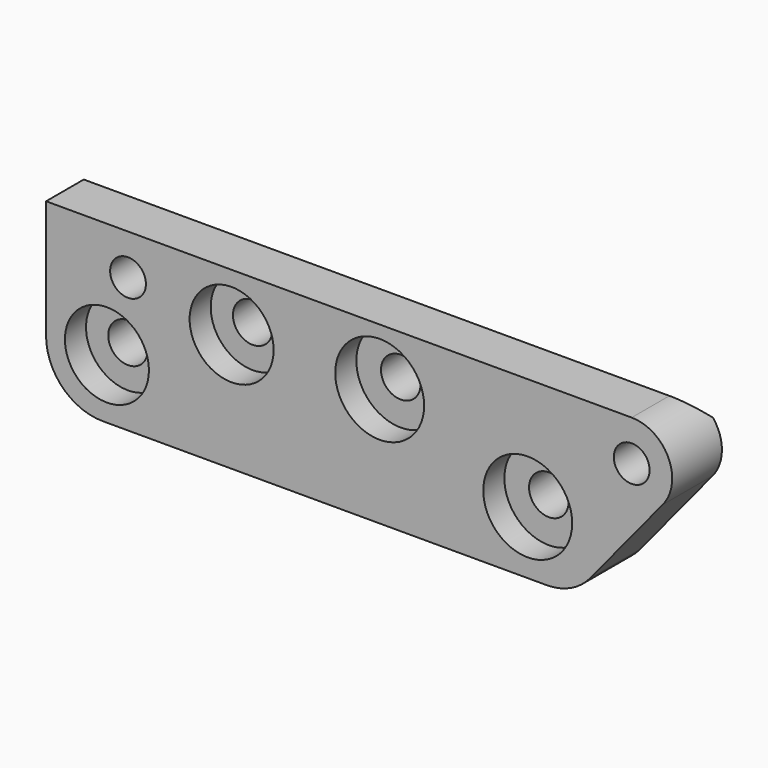
from build123d import *

# Parameters (mm, degrees)
F0_R        = 5.25
F0_R_2      = 4.75
F1_DEPTH    = 16.5
F2_R        = 11.15
F2_R_2      = 11.7991480977
F3_DEPTH    = 7
F4_R        = 15
F5_R        = 15
F6_T1_DEPTH = 176.0234639037


# Not quite as in the source:
# - a fillet or chamfer that OpenCascade refuses, or shapes differently, is made with other operations: its cross-section is extruded or revolved along the edge and cut away or added


with BuildPart() as f1:
    # F0 (on Front) → F1 (new body)
    with BuildSketch(Plane.XZ):
        with BuildLine():
            Line((28.7001559958, 61.0160396297), (-111.2998440042, 61.0160396297))
            Line((-111.2998440042, 61.0160396297), (-111.2998440042, 14.5160396297))
            Line((-111.2998440042, 14.5160396297), (28.7001559958, 14.5160396297))
            Line((28.7001559958, 14.5160396297), (52.362193456, 43.3288254373))
            ThreePointArc((52.362193456, 43.3288254373), (53.9004778512, 54.793039046), (44.1501559958, 61.0160396297))
            Line((44.1501559958, 61.0160396297), (28.7001559958, 61.0160396297))
        make_face()
        with Locations((-95.1498440042, 30.3660396297)):
            Circle(F0_R, mode=Mode.SUBTRACT)
        with Locations((16.5501559958, 31.1660396297)):
            Circle(F0_R, mode=Mode.SUBTRACT)
        with Locations((-62.0498440042, 45.8660396297)):
            Circle(F0_R, mode=Mode.SUBTRACT)
        with Locations((-89.5498440042, 50.2660396297)):
            Circle(F0_R_2, mode=Mode.SUBTRACT)
        with Locations((-22.7498440042, 45.8660396297)):
            Circle(F0_R, mode=Mode.SUBTRACT)
        with Locations((44.1501559958, 50.2660396297)):
            Circle(F0_R_2, mode=Mode.SUBTRACT)
    extrude(amount=F1_DEPTH)

    # F2 (on face) → F3 (cut)
    with BuildSketch(Plane.XZ.offset(16.5)):
        with Locations((-95.1498440042, 30.3660396297)):
            Circle(F2_R)
        with Locations((-62.0498440042, 45.8660396297)):
            Circle(F2_R)
        with Locations((-22.7498440042, 45.8660396297)):
            Circle(F2_R_2)
        with Locations((16.5501559958, 31.1660396297)):
            Circle(F2_R_2)
    extrude(amount=-F3_DEPTH, mode=Mode.SUBTRACT)

    # F4
    f4_edges = [f1.edges().sort_by_distance(p)[0] for p in [
        (28.700156, -8.25, 14.51604),
    ]]
    fillet(f4_edges, radius=F4_R)

    # F5
    f5_edges = [f1.edges().sort_by_distance(p)[0] for p in [
        (-111.299844, -8.25, 14.51604),
    ]]
    fillet(f5_edges, radius=F5_R)

    # F6: chamfer of 4 on 1 edges, made by hand

    # F6_s2 → F6_t1 (cut)
    with BuildSketch(Plane.YZ.offset(-121.5865759561)):
        Polygon((0, 57.0160396297), (-4, 61.0160396297), (0, 61.0160396297), align=None)
    extrude(amount=F6_T1_DEPTH, mode=Mode.SUBTRACT)


solid = f1.part
